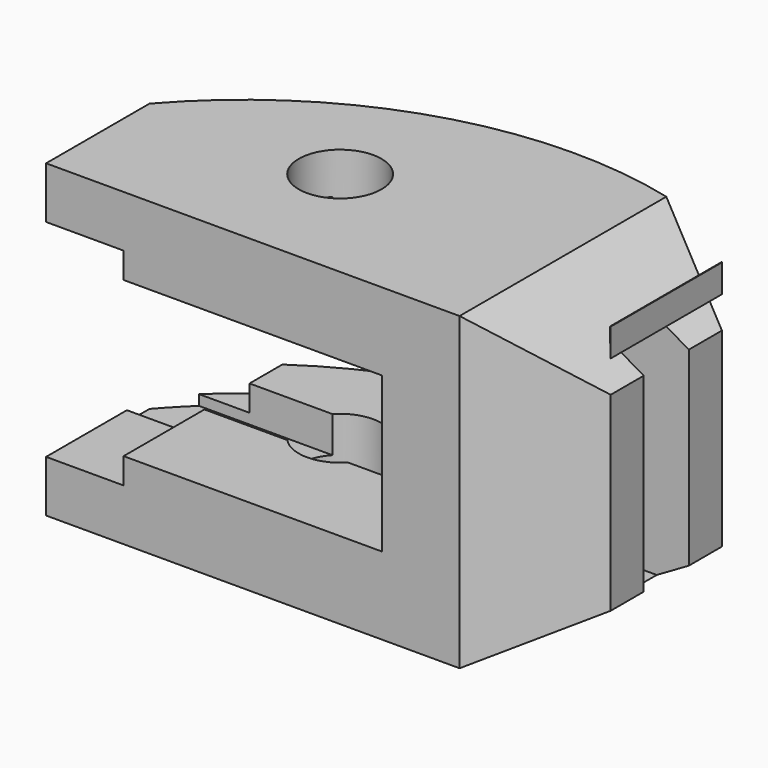
from build123d import *

# Parameters (mm, degrees)
F0_R     = 8
F1_DEPTH = 60
F2_W     = 10.9059892324
F2_H     = 44
F3_DEPTH = 100.001
F5_DEPTH = 52.4578990422


# Not quite as in the source:
# - a feature names something its author has since deleted; it is built from what else it names


with BuildPart() as f1:
    # F0 (on Top) → F1 (new body)
    with BuildSketch(Plane.XY):
        with BuildLine():
            Line((19.6740309507, 27.5431009578), (19.6740309507, 77.5431009578))
            ThreePointArc((19.6740309507, 77.5431009578), (-23.8619994509, 76.3583982428), (-60.3259690493, 52.5431009578))
            Line((-60.3259690493, 52.5431009578), (-60.3259690493, 27.5431009578))
            Line((-60.3259690493, 27.5431009578), (19.6740309507, 27.5431009578))
        make_face()
        with Locations((-23.4298054129, 52.5431009578)):
            Circle(F0_R, mode=Mode.SUBTRACT)
        Polygon((39.6740309507, 65.996095574), (19.6740309507, 77.5431009578), (19.6740309507, 27.5431009578), (39.6740309507, 39.0901063416), align=None)
    extrude(amount=F1_DEPTH)

    # F2 (on face) → F3 (cut, through all)
    with BuildSketch(Plane.YZ.offset(39.6740309507)):
        with Locations((52.5431009578, 30)):
            Rectangle(F2_W, F2_H)
    extrude(amount=-F3_DEPTH, mode=Mode.SUBTRACT)

    # F4 (on face) → F5 (cut, through all)
    with BuildSketch(Plane.XZ.offset(-27.5431009578)):
        Polygon((-60.3259690493, 50), (-60.3259690493, 10), (-45.3259690493, 10), (-45.3259690493, 15), (4.6740309507, 15), (4.6740309507, 30), (4.6740309507, 45), (-45.3259690493, 45), (-45.3259690493, 50), align=None)
        Polygon((39.5541042089, 60), (19.6740309507, 60), (39.8124977946, 48.3188093081), align=None)
        Polygon((39.8124977946, 11.6811906919), (19.6740309507, 0), (39.8124977946, 0), align=None)
    extrude(amount=-F5_DEPTH, mode=Mode.SUBTRACT)


solid = f1.part
